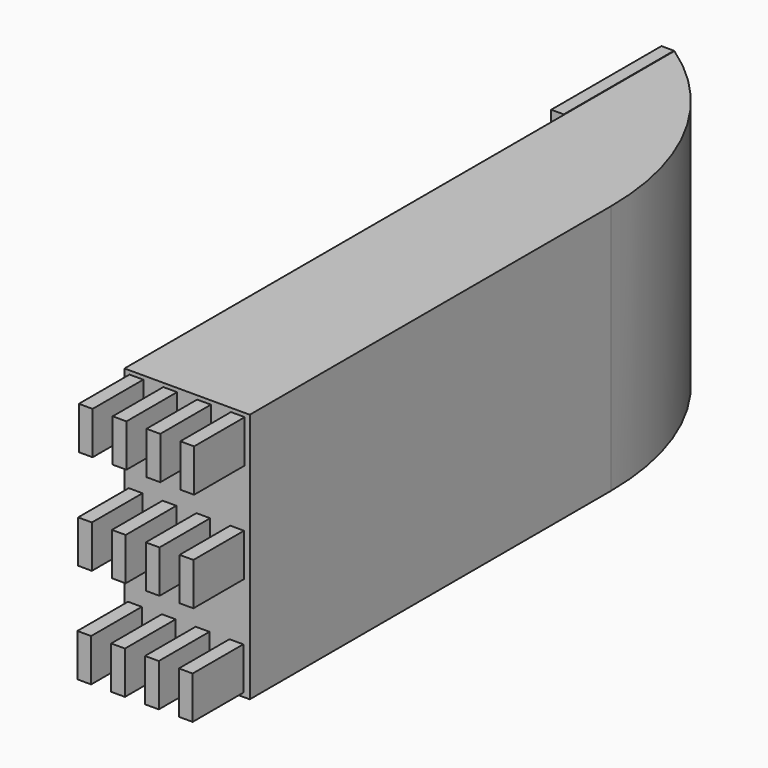
from build123d import *

# Parameters (mm, degrees)
F0_W        = 10
F0_H        = 20
F1_DEPTH    = 25
F3_W        = 30
F3_H        = 20
F4_DEPTH    = 10
F5_T1_DEPTH = 114.1408313715
F6_W        = 11
F6_H        = 20
F7_DEPTH    = 1
F8_W        = 1.1
F8_H        = 3.4004326878
F9_DEPTH    = 5.0529


# Not quite as in the source:
# - a fillet or chamfer that OpenCascade refuses, or shapes differently, is made with other operations: its cross-section is extruded or revolved along the edge and cut away or added


with BuildPart() as f1:
    # F0 (on Front) → F1 (new body)
    with BuildSketch(Plane.XZ):
        Rectangle(F0_W, F0_H)
    extrude(amount=-F1_DEPTH)

    # F3 (on face) → F4 (join)
    with BuildSketch(Plane(origin=(-5, 0, 0), x_dir=(0, -1, 0), z_dir=(-1, 0, 0))):
        with Locations((-39.8661582013, 0)):
            Rectangle(F3_W, F3_H)
    extrude(amount=-F4_DEPTH)

    # F5: fillet of radius 22.7249922626 on 1 edges, made by hand

    # F5_s2 → F5_t1 (cut)
    with BuildSketch(Plane.XY.offset(-57.0704156857)):
        with BuildLine():
            ThreePointArc((-5, 54.8661582013), (2.3448934377, 46.697492915), (5, 36.037991927))
            Line((5, 36.037991927), (5, 54.8661582013))
            Line((5, 54.8661582013), (-5, 54.8661582013))
        make_face()
    extrude(amount=F5_T1_DEPTH, mode=Mode.SUBTRACT)

    # F6 (on face) → F7 (join)
    with BuildSketch(Plane(origin=(-5, 0, 0), x_dir=(0, -1, 0), z_dir=(-1, 0, 0))):
        with Locations((-49.3244222254, 0.0391426826)):
            Rectangle(F6_W, F6_H)
    extrude(amount=F7_DEPTH)

    # F8 (on face) → F9 (join)
    with BuildSketch(Plane.XZ):
        with Locations((-4.05, 7.9997836561)):
            Rectangle(F8_W, F8_H)
        with Locations((-1.35, 7.9997836561)):
            Rectangle(F8_W, F8_H)
        with Locations((1.35, 7.9997836561)):
            Rectangle(F8_W, F8_H)
        with Locations((4.05, 7.9997836561)):
            Rectangle(F8_W, F8_H)
        with Locations((-4.1088341387, 0)):
            Rectangle(F8_W, F8_H)
        with Locations((-4.1676682773, -7.9997836561)):
            Rectangle(F8_W, F8_H)
        with Locations((-1.4088339935, 1.97401e-05)):
            Rectangle(F8_W, F8_H)
        with Locations((-1.467667987, -7.9997441759)):
            Rectangle(F8_W, F8_H)
        with Locations((1.2911689242, 0.0004164637)):
            Rectangle(F8_W, F8_H)
        with Locations((1.2323378484, -7.9989507287)):
            Rectangle(F8_W, F8_H)
        with Locations((3.9911658613, 0)):
            Rectangle(F8_W, F8_H)
        with Locations((3.9323317227, -7.9997836561)):
            Rectangle(F8_W, F8_H)
    extrude(amount=F9_DEPTH)


solid = f1.part
